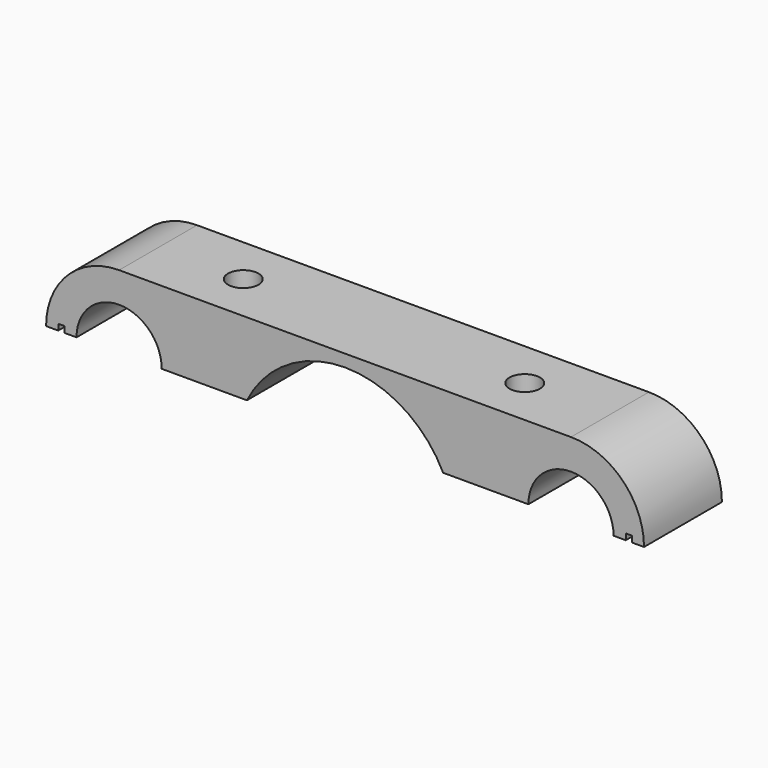
from build123d import *

# Parameters (mm, degrees)
F1_DEPTH = 8
F3_R     = 11.99999
F4_D     = 5
F5_W     = 1
F5_H     = 16
F6_DEPTH = 1


# Not quite as in the source:
# - a fillet or chamfer is up to 0.001 mm smaller than in the source, because OpenCascade refuses the exact size


with BuildPart() as f1:
    # F0 (on Front) → F1 (new body, symmetric)
    with BuildSketch(Plane.XZ):
        with BuildLine():
            Line((-38.25, -6), (-33.25, -6))
            ThreePointArc((-33.25, -6), (-26.25, 1), (-19.25, -6))
            Line((-19.25, -6), (-5.2495154966, -6))
            ThreePointArc((-5.2495154966, -6), (10.875, 4), (26.9995154966, -6))
            Line((26.9995154966, -6), (41, -6))
            ThreePointArc((41, -6), (48, 1), (55, -6))
            Line((55, -6), (60, -6))
            Line((60, -6), (60, 6))
            Line((60, 6), (-38.25, 6))
            Line((-38.25, 6), (-38.25, -6))
        make_face()
    extrude(amount=F1_DEPTH, both=True)

    # F3 (radius 12 in the source; OpenCascade refuses exactly that, so slightly less here)
    f3_edges = [f1.edges().sort_by_distance(p)[0] for p in [
        (-38.25, 0, 6),
        (60, 0, 6),
    ]]
    fillet(f3_edges, radius=F3_R)

    # F4 (through all)
    with Locations(Plane.XY.offset(6)):
        with Locations((-12.25, 0), (34, 0)):
            Hole(F4_D / 2)

    # F5 (on face) → F6 (cut)
    with BuildSketch(Plane(origin=(0, 0, -6), x_dir=(1, 0, 0), z_dir=(0, 0, -1))):
        with Locations((-35.75, 0)):
            Rectangle(F5_W, F5_H)
        with Locations((57.5, 0)):
            Rectangle(F5_W, F5_H)
    extrude(amount=-F6_DEPTH, mode=Mode.SUBTRACT)


solid = f1.part
